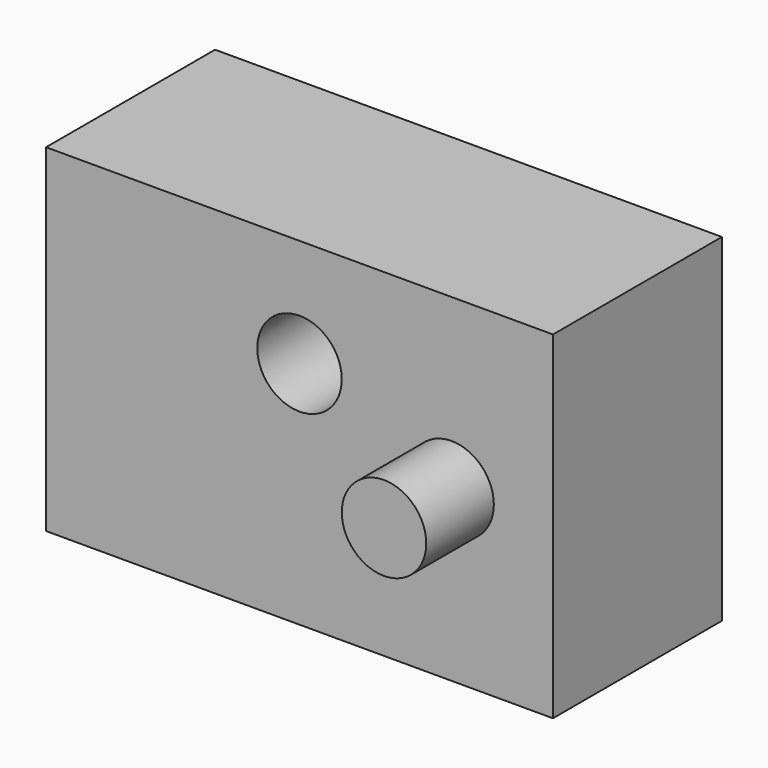
from build123d import *

# Parameters (mm, degrees)
F0_W     = 60
F0_H     = 40
F1_DEPTH = 12.5
F2_R     = 5
F3_DEPTH = 10
F4_R     = 5
F5_DEPTH = 25


# Not quite as in the source:
# - a feature names something its author has since deleted; it is built from what else it names


with BuildPart() as f1:
    # F0 (on Front) → F1 (new body, symmetric)
    with BuildSketch(Plane.XZ):
        Rectangle(F0_W, F0_H)
    extrude(amount=F1_DEPTH, both=True)

    # F2 (on face) → F3 (join)
    with BuildSketch(Plane.XZ.offset(12.5)):
        with Locations((18, 0)):
            Circle(F2_R)
    extrude(amount=F3_DEPTH)

    # F4 (on face) → F5 (cut)
    with BuildSketch(Plane.XZ.offset(12.5)):
        with Locations((0, 7.2016329505)):
            Circle(F4_R)
    extrude(amount=-F5_DEPTH, mode=Mode.SUBTRACT)


solid = f1.part
